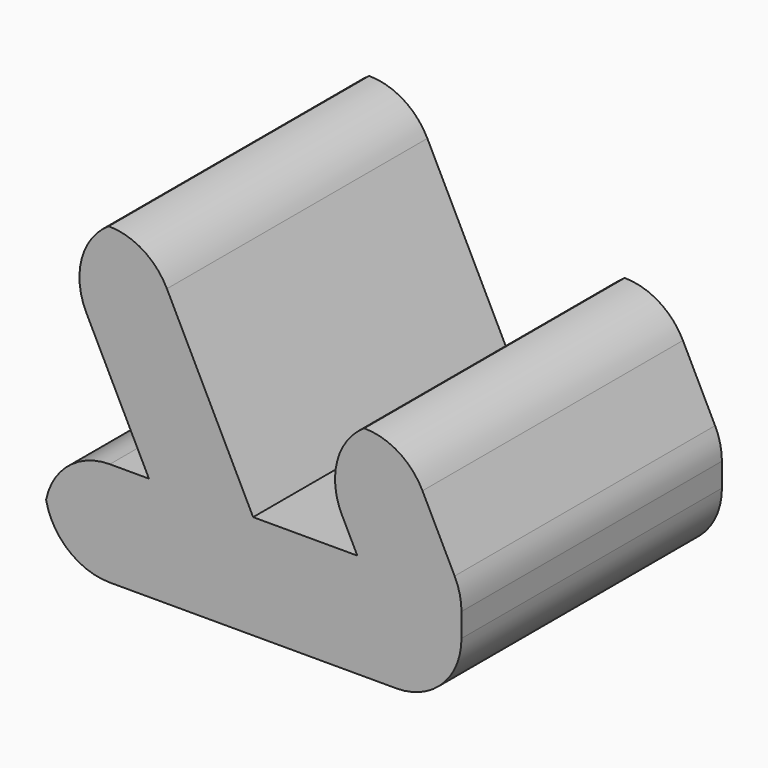
from build123d import *

# Parameters (mm, degrees)
F1_DEPTH    = 25
F2_R        = 5
F3_T1_DEPTH = 60.7481164893
F3_T3_DEPTH = 50
F4_R        = 5


# Not quite as in the source:
# - a fillet or chamfer that OpenCascade refuses, or shapes differently, is made with other operations: its cross-section is extruded or revolved along the edge and cut away or added


with BuildPart() as f1:
    # F0 (on Front) → F1 (new body)
    with BuildSketch(Plane.XZ):
        Polygon((-16, -4), (16, -4), (16, 4), (8, 4), (0, 4), (-8, 4), (-16, 4), align=None)
        Polygon((8, 4), (16, 4), (11.6250231628, 12.7824456607), (3.6250231628, 12.7824456607), align=None)
        Polygon((-16, 20.0594142323), (-8, 4), (0, 4), (-8, 20.0594142323), align=None)
    extrude(amount=F1_DEPTH)

    # F2
    f2_edges = [f1.edges().sort_by_distance(p)[0] for p in [
        (-8, -12.5, 20.059414),
        (11.625023, -12.5, 12.782446),
        (16, -12.5, 4),
    ]]
    fillet(f2_edges, radius=F2_R)

    # F3: fillet of radius 5 on 4 edges, made by hand

    # F3_s2 → F3_t1 (cut)
    with BuildSketch(Plane.XZ.offset(-17.8740582446)):
        with BuildLine():
            ThreePointArc((8.529734301, 12.7824456607), (6.4591533037, 9.9078621452), (6.812957963, 6.3828999728))
            Line((6.812957963, 6.3828999728), (3.6250231628, 12.7824456607))
            Line((3.6250231628, 12.7824456607), (8.529734301, 12.7824456607))
        make_face()
        with BuildLine():
            ThreePointArc((-12.8120651998, 13.6598685445), (-13.1658698591, 17.1848307168), (-11.0952888618, 20.0594142323))
            Line((-11.0952888618, 20.0594142323), (-16, 20.0594142323))
            Line((-16, 20.0594142323), (-12.8120651998, 13.6598685445))
        make_face()
    extrude(amount=F3_T1_DEPTH, mode=Mode.SUBTRACT)

    # F3_s4 → F3_t3 (cut)
    with BuildSketch(Plane.XZ.offset(-12.5)):
        with BuildLine():
            ThreePointArc((-16, -1), (-14.5355339059, 2.5355339059), (-11, 4))
            Line((-11, 4), (-16, 4))
            Line((-16, 4), (-16, -1))
        make_face()
        with BuildLine():
            ThreePointArc((-11, -4), (-14.5355339059, -2.5355339059), (-16, 1))
            Line((-16, 1), (-16, -4))
            Line((-16, -4), (-11, -4))
        make_face()
    extrude(amount=F3_T3_DEPTH, mode=Mode.SUBTRACT)

    # F4
    f4_edges = [f1.edges().sort_by_distance(p)[0] for p in [
        (16, -12.5, -4),
    ]]
    fillet(f4_edges, radius=F4_R)


solid = f1.part
